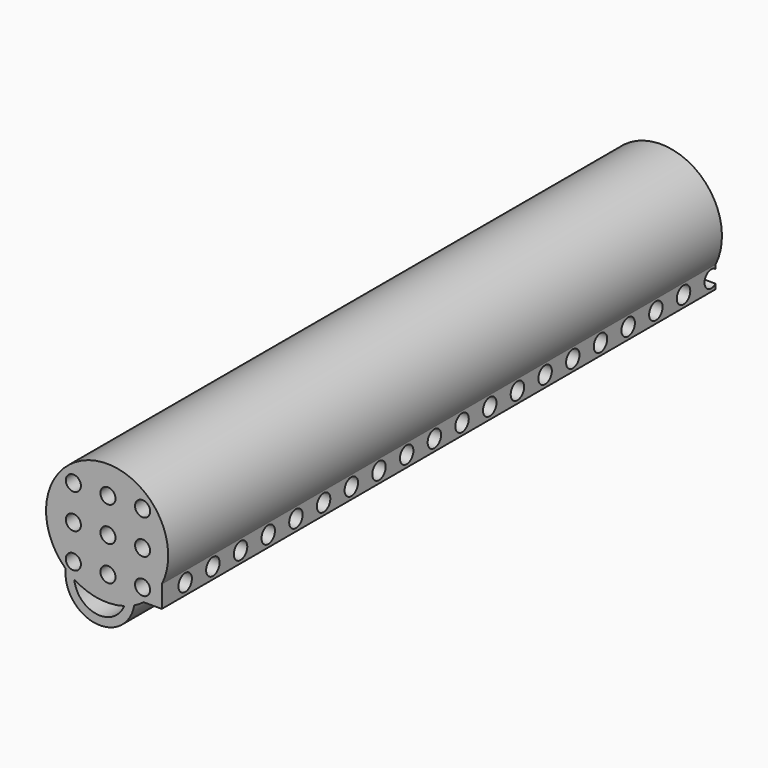
from build123d import *

# Parameters (mm, degrees)
F0_R      = 25.4
F1_DEPTH  = 508
F2_R      = 19.05
F3_DEPTH  = 508
F4_W      = 24.185795337
F4_H      = 19.6861149743
F5_DEPTH  = 254
F6_R      = 2.5527
F7_DEPTH  = 254
F8_W      = 61.5894217044
F8_H      = 30.7947099209
F9_DEPTH  = 508
F10_R     = 8.5769921684
F11_DEPTH = 508
F12_R     = 44.8321943463
F13_DEPTH = 508
F14_R     = 5.5398710305
F15_DEPTH = 762
F16_R     = 6.1676361256
F17_DEPTH = 508
F18_R     = 8.0611357012
F20_DEPTH = 508


# Not quite as in the source:
# - the program builds the solid bodies; features that only make, move or delete a surface that nothing else refers to are left out


with BuildPart() as f1:
    # F0 (on Front) → F1 (new body)
    with BuildSketch(Plane.XZ):
        Circle(F0_R)
    extrude(amount=F1_DEPTH)

    # F2 (on face) → F3 (cut)
    with BuildSketch(Plane.XZ.offset(508)):
        Circle(F2_R)
    extrude(amount=-F3_DEPTH, mode=Mode.SUBTRACT)

    # F8 (on Front) → F9 (join)
    with BuildSketch(Plane.XZ):
        with Locations((14.4833577797, 15.3973549604)):
            Rectangle(F8_W, F8_H)
    extrude(amount=F9_DEPTH)

    # F10 (on face) → F11 (cut)
    with BuildSketch(Plane.XY.offset(30.7947099209)):
        with Locations((32.5780686319, -495.3)):
            Circle(F10_R)
        with Locations((32.5780686319, -469.9)):
            Circle(F10_R)
        with Locations((32.5780686319, -444.5)):
            Circle(F10_R)
        with Locations((32.5780686319, -419.1)):
            Circle(F10_R)
        with Locations((32.5780686319, -393.7)):
            Circle(F10_R)
        with Locations((32.5780686319, -368.3)):
            Circle(F10_R)
        with Locations((32.5780686319, -342.9)):
            Circle(F10_R)
        with Locations((32.5780686319, -317.5)):
            Circle(F10_R)
        with Locations((32.5780686319, -292.1)):
            Circle(F10_R)
        with Locations((32.5780686319, -266.7)):
            Circle(F10_R)
        with Locations((32.5780686319, -241.3)):
            Circle(F10_R)
        with Locations((32.5780686319, -215.9)):
            Circle(F10_R)
        with Locations((32.5780686319, -190.5)):
            Circle(F10_R)
        with Locations((32.5780686319, -165.1)):
            Circle(F10_R)
        with Locations((32.5780686319, -139.7)):
            Circle(F10_R)
        with Locations((32.5780686319, -114.3)):
            Circle(F10_R)
        with Locations((32.5780686319, -88.9)):
            Circle(F10_R)
        with Locations((32.5780686319, -63.5)):
            Circle(F10_R)
        with Locations((32.5780686319, -38.1)):
            Circle(F10_R)
        with Locations((32.5780686319, -12.7)):
            Circle(F10_R)
        with Locations((7.1780686319, -469.9)):
            Circle(F10_R)
        with Locations((7.1780686319, -444.5)):
            Circle(F10_R)
        with Locations((7.1780686319, -419.1)):
            Circle(F10_R)
        with Locations((7.1780686319, -393.7)):
            Circle(F10_R)
        with Locations((7.1780686319, -368.3)):
            Circle(F10_R)
        with Locations((7.1780686319, -342.9)):
            Circle(F10_R)
        with Locations((7.1780686319, -317.5)):
            Circle(F10_R)
        with Locations((7.1780686319, -292.1)):
            Circle(F10_R)
        with Locations((7.1780686319, -266.7)):
            Circle(F10_R)
        with Locations((7.1780686319, -241.3)):
            Circle(F10_R)
        with Locations((7.1780686319, -215.9)):
            Circle(F10_R)
        with Locations((7.1780686319, -190.5)):
            Circle(F10_R)
        with Locations((7.1780686319, -165.1)):
            Circle(F10_R)
        with Locations((7.1780686319, -139.7)):
            Circle(F10_R)
        with Locations((7.1780686319, -114.3)):
            Circle(F10_R)
        with Locations((7.1780686319, -88.9)):
            Circle(F10_R)
        with Locations((7.1780686319, -63.5)):
            Circle(F10_R)
        with Locations((7.1780686319, -38.1)):
            Circle(F10_R)
        with Locations((7.1780686319, -12.7)):
            Circle(F10_R)
    extrude(amount=-F11_DEPTH, mode=Mode.SUBTRACT)

    # F12 (on Front) → F13 (join)
    with BuildSketch(Plane.XZ):
        with Locations((5.1357760094, 35.9504371881)):
            Circle(F12_R)
    extrude(amount=F13_DEPTH)

    # F14 (on face) → F15 (cut)
    with BuildSketch(Plane.XZ.offset(508)):
        with Locations((-19.6441602525, 60.2015365373)):
            Circle(F14_R)
        with Locations((-19.6441602525, 34.8015365373)):
            Circle(F14_R)
        with Locations((-19.6441602525, 9.4015365373)):
            Circle(F14_R)
        with Locations((5.7558397475, 60.2015365373)):
            Circle(F14_R)
        with Locations((5.7558397475, 34.8015365373)):
            Circle(F14_R)
        with Locations((5.7558397475, 9.4015365373)):
            Circle(F14_R)
        with Locations((31.1558397475, 60.2015365373)):
            Circle(F14_R)
        with Locations((31.1558397475, 34.8015365373)):
            Circle(F14_R)
        with Locations((31.1558397475, 9.4015365373)):
            Circle(F14_R)
    extrude(amount=-F15_DEPTH, mode=Mode.SUBTRACT)

    # F16 (on face) → F17 (cut)
    with BuildSketch(Plane.YZ.offset(45.2780686319)):
        with Locations((-486.5653300281, 8.3674215613)):
            Circle(F16_R)
        with Locations((-461.1653300281, 8.3674215613)):
            Circle(F16_R)
        with Locations((-435.7653300281, 8.3674215613)):
            Circle(F16_R)
        with Locations((-410.3653300281, 8.3674215613)):
            Circle(F16_R)
        with Locations((-384.9653300281, 8.3674215613)):
            Circle(F16_R)
        with Locations((-359.5653300281, 8.3674215613)):
            Circle(F16_R)
        with Locations((-334.1653300281, 8.3674215613)):
            Circle(F16_R)
        with Locations((-308.7653300281, 8.3674215613)):
            Circle(F16_R)
        with Locations((-283.3653300281, 8.3674215613)):
            Circle(F16_R)
        with Locations((-257.9653300281, 8.3674215613)):
            Circle(F16_R)
        with Locations((-232.5653300281, 8.3674215613)):
            Circle(F16_R)
        with Locations((-207.1653300281, 8.3674215613)):
            Circle(F16_R)
        with Locations((-181.7653300281, 8.3674215613)):
            Circle(F16_R)
        with Locations((-156.3653300281, 8.3674215613)):
            Circle(F16_R)
        with Locations((-130.9653300281, 8.3674215613)):
            Circle(F16_R)
        with Locations((-105.5653300281, 8.3674215613)):
            Circle(F16_R)
        with Locations((-80.1653300281, 8.3674215613)):
            Circle(F16_R)
        with Locations((-54.7653300281, 8.3674215613)):
            Circle(F16_R)
        with Locations((-29.3653300281, 8.3674215613)):
            Circle(F16_R)
        with Locations((-3.9653300281, 8.3674215613)):
            Circle(F16_R)
    extrude(amount=-F17_DEPTH, mode=Mode.SUBTRACT)


with BuildPart() as f5:
    # F4 (on Front) → F5 (new body)
    with BuildSketch(Plane.XZ):
        with Locations((-53.714973852, 16.1707377993)):
            Rectangle(F4_W, F4_H)
    extrude(amount=F5_DEPTH)

    # F6 (on face) → F7 (cut)
    with BuildSketch(Plane(origin=(0, 0, 6.3276803121), x_dir=(1, 0, 0), z_dir=(0, 0, -1))):
        with Locations((-53.1078715205, 241.3)):
            Circle(F6_R)
        with Locations((-53.1078715205, 215.9)):
            Circle(F6_R)
        with Locations((-53.1078715205, 190.5)):
            Circle(F6_R)
        with Locations((-53.1078715205, 165.1)):
            Circle(F6_R)
        with Locations((-53.1078715205, 139.7)):
            Circle(F6_R)
        with Locations((-53.1078715205, 114.3)):
            Circle(F6_R)
        with Locations((-53.1078715205, 88.9)):
            Circle(F6_R)
        with Locations((-53.1078715205, 63.5)):
            Circle(F6_R)
        with Locations((-53.1078715205, 38.1)):
            Circle(F6_R)
        with Locations((-53.1078715205, 12.7)):
            Circle(F6_R)
    extrude(amount=-F7_DEPTH, mode=Mode.SUBTRACT)

    # F18 (on face) → F20 (cut)
    with BuildSketch(Plane(origin=(-65.8078715205, 0, 0), x_dir=(0, -1, 0), z_dir=(-1, 0, 0))):
        with Locations((244.1448, 16.1707377993)):
            Circle(F18_R)
        with Locations((218.7448, 16.1707377993)):
            Circle(F18_R)
        with Locations((193.3448, 16.1707377993)):
            Circle(F18_R)
        with Locations((167.9448, 16.1707377993)):
            Circle(F18_R)
        with Locations((142.5448, 16.1707377993)):
            Circle(F18_R)
        with Locations((117.1448, 16.1707377993)):
            Circle(F18_R)
        with Locations((91.7448, 16.1707377993)):
            Circle(F18_R)
        with Locations((66.3448, 16.1707377993)):
            Circle(F18_R)
        with Locations((40.9448, 16.1707377993)):
            Circle(F18_R)
        with Locations((15.5448, 16.1707377993)):
            Circle(F18_R)
        with Locations((-9.8552, 16.1707377993)):
            Circle(F18_R)
        with Locations((-35.2552, 16.1707377993)):
            Circle(F18_R)
        with Locations((-60.6552, 16.1707377993)):
            Circle(F18_R)
        with Locations((-86.0552, 16.1707377993)):
            Circle(F18_R)
        with Locations((-111.4552, 16.1707377993)):
            Circle(F18_R)
        with Locations((-136.8552, 16.1707377993)):
            Circle(F18_R)
        with Locations((-162.2552, 16.1707377993)):
            Circle(F18_R)
        with Locations((-187.6552, 16.1707377993)):
            Circle(F18_R)
        with Locations((-213.0552, 16.1707377993)):
            Circle(F18_R)
        with Locations((-238.4552, 16.1707377993)):
            Circle(F18_R)
    extrude(amount=-F20_DEPTH, mode=Mode.SUBTRACT)


solid = Compound([f1.part, f5.part])
